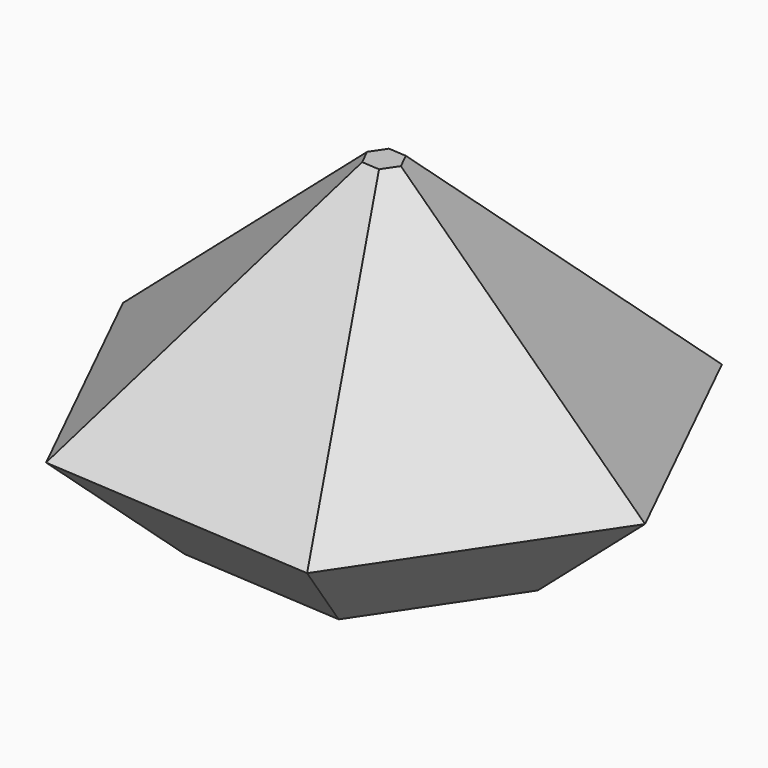
from build123d import *

# Parameters (mm, degrees)
F1_DEPTH     = 38.1
F2_SIZE      = 22.86
F3_W         = 104.742500931
F3_H         = 73.319750838
F4_DEPTH     = 38.1
F5_T1_DEPTH  = 93.1636902777
F5_T3_DEPTH  = 93.1636902777
F5_T5_DEPTH  = 93.1636902777
F5_T7_DEPTH  = 93.1636902777
F5_T9_DEPTH  = 93.1636902777
F5_T11_DEPTH = 93.1636902777


# Not quite as in the source:
# - a fillet or chamfer that OpenCascade refuses, or shapes differently, is made with other operations: its cross-section is extruded or revolved along the edge and cut away or added


with BuildPart() as f1:
    # F0 (on Top) → F1 (new body, symmetric)
    with BuildSketch(Plane.XY):
        Polygon((15.5198623998, 23.1162996964), (-12.2593715787, 24.9987449497), (-27.7792339785, 1.8824452533), (-15.5198623998, -23.1162996964), (12.2593715787, -24.9987449497), (27.7792339785, -1.8824452533), align=None)
    extrude(amount=F1_DEPTH, both=True)

    # F2
    f2_edges = [f1.edges().sort_by_distance(p)[0] for p in [
        (21.649548, 10.616927, 38.1),
        (1.630245, 24.057522, 38.1),
        (-20.019303, 13.440595, 38.1),
        (-21.649548, -10.616927, 38.1),
        (-1.630245, -24.057522, 38.1),
        (20.019303, -13.440595, 38.1),
    ]]
    chamfer(f2_edges, length=F2_SIZE)

    # F3 (on Right) → F4 (cut, symmetric)
    with BuildSketch(Plane.YZ):
        with Locations((-5.571493879, -24.6362821199)):
            Rectangle(F3_W, F3_H)
    extrude(amount=F4_DEPTH, both=True, mode=Mode.SUBTRACT)

    # F5: chamfer of 12.7 on 6 edges, made by hand

    # F5_s2 → F5_t1 (cut)
    with BuildSketch(Plane(origin=(-20.5101939484, 41.8234412828, 0), x_dir=(0, 0, 1), z_dir=(0.4403044553, -0.8978485322, 0))):
        Polygon((24.7235932991, -24.1126954201), (12.0235932991, -11.4126954201), (12.0235932991, -24.1126954201), align=None)
    extrude(amount=F5_T1_DEPTH, mode=Mode.SUBTRACT)

    # F5_s4 → F5_t3 (cut)
    with BuildSketch(Plane(origin=(25.9650656504, 38.6740696373, 0), x_dir=(0, 0, 1), z_dir=(-0.55740741, -0.8302391097, 0))):
        Polygon((12.0235932991, -11.4126954201), (24.7235932991, -24.1126954201), (12.0235932991, -24.1126954201), align=None)
    extrude(amount=F5_T3_DEPTH, mode=Mode.SUBTRACT)

    # F5_s6 → F5_t5 (cut)
    with BuildSketch(Plane(origin=(46.4752595988, -3.1493716455, 0), x_dir=(0, 0, 1), z_dir=(-0.9977118652, 0.0676094224, 0))):
        Polygon((12.0235932991, -11.4126954201), (24.7235932991, -24.1126954201), (12.0235932991, -24.1126954201), align=None)
    extrude(amount=F5_T5_DEPTH, mode=Mode.SUBTRACT)

    # F5_s8 → F5_t7 (cut)
    with BuildSketch(Plane(origin=(20.5101939484, -41.8234412828, 0), x_dir=(0, 0, 1), z_dir=(-0.4403044553, 0.8978485322, 0))):
        Polygon((12.0235932991, -11.4126954201), (24.7235932991, -24.1126954201), (12.0235932991, -24.1126954201), align=None)
    extrude(amount=F5_T7_DEPTH, mode=Mode.SUBTRACT)

    # F5_s10 → F5_t9 (cut)
    with BuildSketch(Plane(origin=(-25.9650656504, -38.6740696373, 0), x_dir=(0, 0, 1), z_dir=(0.55740741, 0.8302391097, 0))):
        Polygon((12.0235932991, -11.4126954201), (24.7235932991, -24.1126954201), (12.0235932991, -24.1126954201), align=None)
    extrude(amount=F5_T9_DEPTH, mode=Mode.SUBTRACT)

    # F5_s12 → F5_t11 (cut)
    with BuildSketch(Plane(origin=(-46.4752595988, 3.1493716455, 0), x_dir=(0, 0, 1), z_dir=(0.9977118652, -0.0676094224, 0))):
        Polygon((12.0235932991, -11.4126954201), (24.7235932991, -24.1126954201), (12.0235932991, -24.1126954201), align=None)
    extrude(amount=F5_T11_DEPTH, mode=Mode.SUBTRACT)


solid = f1.part
